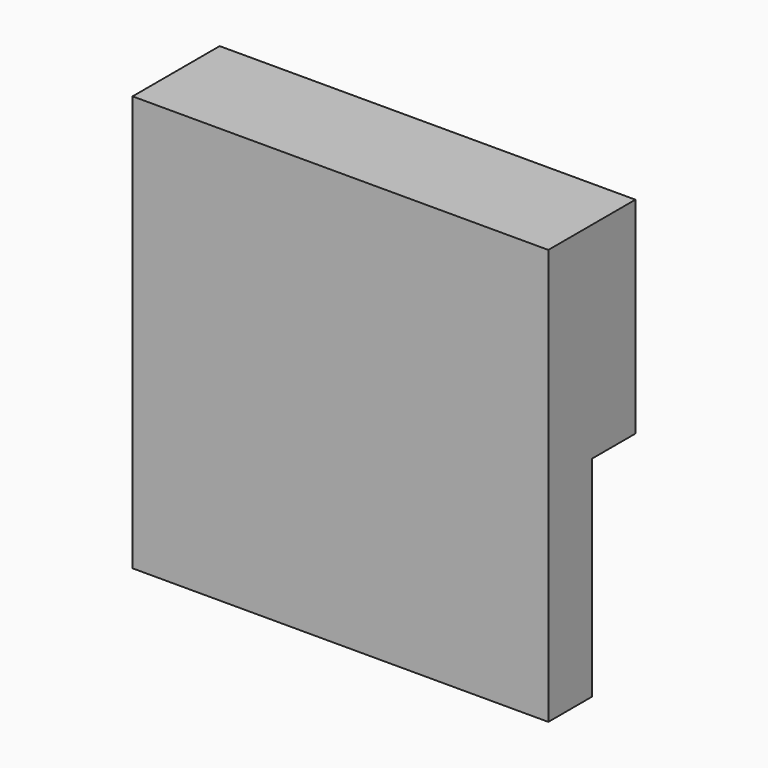
from build123d import *

# Parameters (mm, degrees)
F0_W     = 194.0150633454
F0_H     = 193.9053460956
F1_DEPTH = 25.4
F2_W     = 76.4794424176
F2_H     = 75.5990371108
F2_H_2   = 76.2040093541
F2_W_2   = 74.5813548565
F3_DEPTH = 25.4


with BuildPart() as f1:
    # F0 (on Front) → F1 (new body)
    with BuildSketch(Plane.XZ):
        with Locations((-0.3764815629, -0.8369870484)):
            Rectangle(F0_W, F0_H)
    extrude(amount=F1_DEPTH)

    # F2 (on face) → F3 (join)
    with BuildSketch(Plane(origin=(0, 0, 0), x_dir=(-1, 0, 0), z_dir=(0, 1, 0))):
        with Locations((38.2397212088, 37.7995185554)):
            Rectangle(F2_W, F2_H)
        with Locations((38.2397212088, -38.1020046771)):
            Rectangle(F2_W, F2_H_2)
        with Locations((-37.2906774282, 37.7995185554)):
            Rectangle(F2_W_2, F2_H)
        Polygon((97.3840132356, 0), (76.4794424176, 0), (76.4794424176, -76.2040093541), (0, -76.2040093541), (0, -97.7896600962), (97.3840132356, -97.7896600962), align=None)
        Polygon((76.4794424176, 75.5990371108), (76.4794424176, 0), (97.3840132356, 0), (97.3840132356, 96.1156859994), (-96.6310501099, 96.1156859994), (-96.6310501099, 0), (-74.5813548565, 0), (-74.5813548565, 75.5990371108), (0, 75.5990371108), align=None)
    extrude(amount=F3_DEPTH)


solid = f1.part
